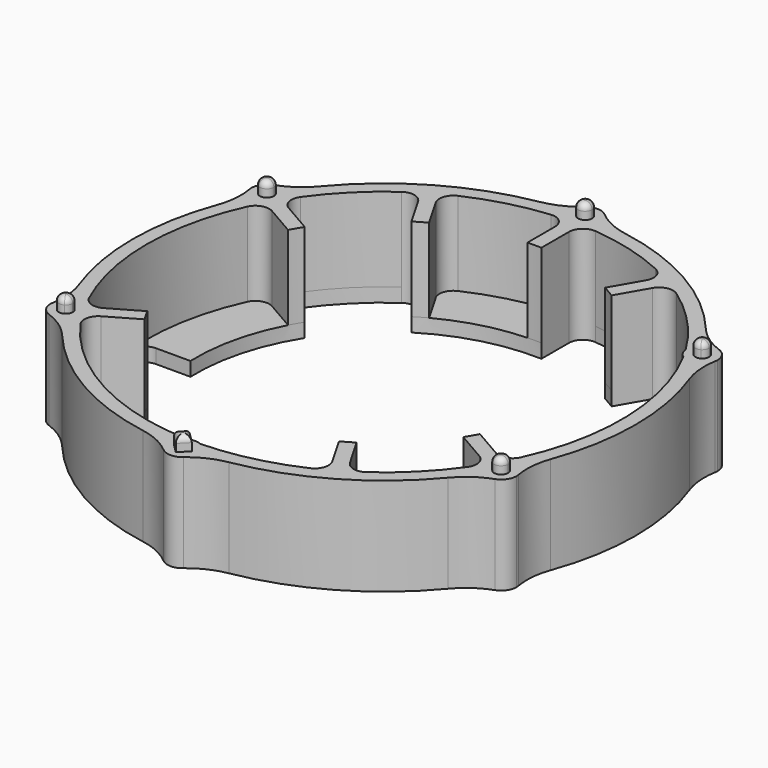
from build123d import *

# Parameters (mm, degrees)
F1_R         = 18
F1_R_2       = 17
F2_DEPTH     = 7
F3_DEPTH     = 7
F4_DEPTH     = 1
F6_DEPTH     = 7
F7_R         = 1
F8_R         = 5
F9_DEPTH     = 8
F10_R        = 0.44999
F11_DEPTH    = 1.8
F12_R        = 13.47
F13_DEPTH    = 1
F14_DEPTH    = 1
F15_T1_DEPTH = 1
F15_T3_DEPTH = 3.7395798703


# Not quite as in the source:
# - a fillet or chamfer that OpenCascade refuses, or shapes differently, is made with other operations: its cross-section is extruded or revolved along the edge and cut away or added
# - a fillet or chamfer is up to 0.001 mm smaller than in the source, because OpenCascade refuses the exact size


with BuildPart() as f2:
    # F1 (on Top) → F2 (new body)
    with BuildSketch(Plane.XY):
        Circle(F1_R)
        Circle(F1_R_2, mode=Mode.SUBTRACT)
    extrude(amount=F2_DEPTH)

    # F0 (on Top) → F3 (join)
    with BuildSketch(Plane.XY):
        with BuildLine():
            Line((-11.4073228059, 7.1633711619), (-14.4660626528, 8.9293354359))
            ThreePointArc((-14.4660626528, 8.9293354359), (-14.7224318643, 8.5), (-14.9660626528, 8.0633100321))
            Line((-14.9660626528, 8.0633100321), (-11.9073228059, 6.2973457581))
            ThreePointArc((-11.9073228059, 6.2973457581), (-11.665362189, 6.735), (-11.4073228059, 7.1633711619))
        make_face()
        with BuildLine():
            Line((7.1633711619, 11.4073228059), (8.9293354359, 14.4660626528))
            ThreePointArc((8.9293354359, 14.4660626528), (8.5, 14.7224318643), (8.0633100321, 14.9660626528))
            Line((8.0633100321, 14.9660626528), (6.2973457581, 11.9073228059))
            ThreePointArc((6.2973457581, 11.9073228059), (6.735, 11.665362189), (7.1633711619, 11.4073228059))
        make_face()
        with BuildLine():
            ThreePointArc((-14.9660626528, -8.0633100321), (-14.7224318643, -8.5), (-14.4660626528, -8.9293354359))
            Line((-14.4660626528, -8.9293354359), (-11.4073228059, -7.1633711619))
            ThreePointArc((-11.4073228059, -7.1633711619), (-11.665362189, -6.735), (-11.9073228059, -6.2973457581))
            Line((-11.9073228059, -6.2973457581), (-14.9660626528, -8.0633100321))
        make_face()
        with BuildLine():
            Line((-6.2973457581, 11.9073228059), (-8.0633100321, 14.9660626528))
            ThreePointArc((-8.0633100321, 14.9660626528), (-8.5, 14.7224318643), (-8.9293354359, 14.4660626528))
            Line((-8.9293354359, 14.4660626528), (-7.1633711619, 11.4073228059))
            ThreePointArc((-7.1633711619, 11.4073228059), (-6.735, 11.665362189), (-6.2973457581, 11.9073228059))
        make_face()
        with BuildLine():
            Line((0.5, 13.46071692), (0.5, 16.992645468))
            ThreePointArc((0.5, 16.992645468), (0, 17), (-0.5, 16.992645468))
            Line((-0.5, 16.992645468), (-0.5, 13.46071692))
            ThreePointArc((-0.5, 13.46071692), (0, 13.47), (0.5, 13.46071692))
        make_face()
        with BuildLine():
            ThreePointArc((14.4660626528, -8.9293354359), (14.7224318643, -8.5), (14.9660626528, -8.0633100321))
            Line((14.9660626528, -8.0633100321), (11.9073228059, -6.2973457581))
            ThreePointArc((11.9073228059, -6.2973457581), (11.665362189, -6.735), (11.4073228059, -7.1633711619))
            Line((11.4073228059, -7.1633711619), (14.4660626528, -8.9293354359))
        make_face()
        with BuildLine():
            ThreePointArc((8.0633100321, -14.9660626528), (8.5, -14.7224318643), (8.9293354359, -14.4660626528))
            Line((8.9293354359, -14.4660626528), (7.1633711619, -11.4073228059))
            ThreePointArc((7.1633711619, -11.4073228059), (6.735, -11.665362189), (6.2973457581, -11.9073228059))
            Line((6.2973457581, -11.9073228059), (8.0633100321, -14.9660626528))
        make_face()
    extrude(amount=F3_DEPTH)

    # F1 (on Top) → F4 (join)
    with BuildSketch(Plane.XY):
        Circle(F1_R)
        Circle(F1_R_2, mode=Mode.SUBTRACT)
        Circle(F1_R_2)
    extrude(amount=F4_DEPTH)

    # F5 (on Top) → F6 (join)
    with BuildSketch(Plane.XY):
        with BuildLine():
            ThreePointArc((-14.4884572681, 9), (-14.6275367743, 9.5353800561), (-15.0096060035, 9.935377578))
            ThreePointArc((-15.0096060035, 9.935377578), (-15.1731450826, 9.6837837802), (-15.3324673166, 9.4294987133))
            ThreePointArc((-15.3324673166, 9.4294987133), (-15.153718855, 9.2469868663), (-15.0884572681, 9))
            ThreePointArc((-15.0884572681, 9), (-15.3354561915, 8.5687338928), (-15.832419089, 8.5635568422))
            ThreePointArc((-15.832419089, 8.5635568422), (-15.9729752997, 8.2984372068), (-16.1090923805, 8.0310113108))
            ThreePointArc((-16.1090923805, 8.0310113108), (-15.0239657375, 8.0558870238), (-14.4884572681, 9))
        make_face()
        with BuildLine():
            ThreePointArc((-15.3324673166, 9.4294987133), (-15.1731450826, 9.6837837802), (-15.0096060035, 9.935377578))
            ThreePointArc((-15.0096060035, 9.935377578), (-16.5410852123, 9.55), (-16.1090923805, 8.0310113108))
            ThreePointArc((-16.1090923805, 8.0310113108), (-15.9729752997, 8.2984372068), (-15.832419089, 8.5635568422))
            ThreePointArc((-15.832419089, 8.5635568422), (-16.02146997, 9.25), (-15.3324673166, 9.4294987133))
        make_face()
        with BuildLine():
            ThreePointArc((-1.099486377, 17.9663888889), (0, 16.9), (1.099486377, 17.9663888889))
            ThreePointArc((1.099486377, 17.9663888889), (0.7998302171, 17.982220987), (0.4999517724, 17.9930555556))
            ThreePointArc((0.4999517724, 17.9930555556), (0, 17.5), (-0.4999517724, 17.9930555556))
            ThreePointArc((-0.4999517724, 17.9930555556), (-0.7998302171, 17.982220987), (-1.099486377, 17.9663888889))
        make_face()
        with BuildLine():
            ThreePointArc((0.4999517724, 17.9930555556), (0.7998302171, 17.982220987), (1.099486377, 17.9663888889))
            ThreePointArc((1.099486377, 17.9663888889), (1.0998715868, 17.9831924823), (1.1, 18))
            ThreePointArc((1.1, 18), (-0.0168075177, 19.0998715868), (-1.099486377, 17.9663888889))
            ThreePointArc((-1.099486377, 17.9663888889), (-0.7998302171, 17.982220987), (-0.4999517724, 17.9930555556))
            ThreePointArc((-0.4999517724, 17.9930555556), (-0.003472306, 18.4999879429), (0.5, 18))
            ThreePointArc((0.5, 18), (0.4999879429, 17.996527694), (0.4999517724, 17.9930555556))
        make_face()
        with BuildLine():
            ThreePointArc((15.832419089, 8.5635568422), (15.9729752997, 8.2984372068), (16.1090923805, 8.0310113108))
            ThreePointArc((16.1090923805, 8.0310113108), (16.5325702443, 8.4355084694), (16.6884572681, 9))
            ThreePointArc((16.6884572681, 9), (16.1238373242, 9.9609204939), (15.0096060035, 9.935377578))
            ThreePointArc((15.0096060035, 9.935377578), (15.1731450826, 9.6837837802), (15.3324673166, 9.4294987133))
            ThreePointArc((15.3324673166, 9.4294987133), (15.8354441344, 9.4347384132), (16.0884572681, 9))
            ThreePointArc((16.0884572681, 9), (16.0197233753, 8.7469989234), (15.832419089, 8.5635568422))
        make_face()
        with BuildLine():
            ThreePointArc((15.0096060035, 9.935377578), (14.635829324, 8.45), (16.1090923805, 8.0310113108))
            ThreePointArc((16.1090923805, 8.0310113108), (15.9729752997, 8.2984372068), (15.832419089, 8.5635568422))
            ThreePointArc((15.832419089, 8.5635568422), (15.1554445662, 8.75), (15.3324673166, 9.4294987133))
            ThreePointArc((15.3324673166, 9.4294987133), (15.1731450826, 9.6837837802), (15.0096060035, 9.935377578))
        make_face()
        with BuildLine():
            ThreePointArc((-15.3324673166, -9.4294987133), (-15.1731450826, -9.6837837802), (-15.0096060035, -9.935377578))
            ThreePointArc((-15.0096060035, -9.935377578), (-14.6275367743, -9.5353800561), (-14.4884572681, -9))
            ThreePointArc((-14.4884572681, -9), (-15.0239657375, -8.0558870238), (-16.1090923805, -8.0310113108))
            ThreePointArc((-16.1090923805, -8.0310113108), (-15.9729752997, -8.2984372068), (-15.832419089, -8.5635568422))
            ThreePointArc((-15.832419089, -8.5635568422), (-15.3354561915, -8.5687338928), (-15.0884572681, -9))
            ThreePointArc((-15.0884572681, -9), (-15.153718855, -9.2469868663), (-15.3324673166, -9.4294987133))
        make_face()
        with BuildLine():
            ThreePointArc((-16.1090923805, -8.0310113108), (-16.5410852123, -9.55), (-15.0096060035, -9.935377578))
            ThreePointArc((-15.0096060035, -9.935377578), (-15.1731450826, -9.6837837802), (-15.3324673166, -9.4294987133))
            ThreePointArc((-15.3324673166, -9.4294987133), (-16.02146997, -9.25), (-15.832419089, -8.5635568422))
            ThreePointArc((-15.832419089, -8.5635568422), (-15.9729752997, -8.2984372068), (-16.1090923805, -8.0310113108))
        make_face()
        with BuildLine():
            ThreePointArc((0.6255239257, -17.9891278226), (0.8625800837, -17.9793202207), (1.099486377, -17.9663888889))
            ThreePointArc((1.099486377, -17.9663888889), (0, -16.9), (-1.099486377, -17.9663888889))
            ThreePointArc((-1.099486377, -17.9663888889), (-0.8625800837, -17.9793202207), (-0.6255239257, -17.9891278226))
            Line((-0.6255239257, -17.9891278226), (0, -17.3636038969))
            Line((0, -17.3636038969), (0.6255239257, -17.9891278226))
        make_face()
        with BuildLine():
            ThreePointArc((1.1, -18), (1.0998715868, -17.9831924823), (1.099486377, -17.9663888889))
            ThreePointArc((1.099486377, -17.9663888889), (0.8625800837, -17.9793202207), (0.6255239257, -17.9891278226))
            Line((0.6255239257, -17.9891278226), (0.6363961031, -18))
            Line((0.6363961031, -18), (0, -18.6363961031))
            Line((0, -18.6363961031), (-0.6363961031, -18))
            Line((-0.6363961031, -18), (-0.6255239257, -17.9891278226))
            ThreePointArc((-0.6255239257, -17.9891278226), (-0.8625800837, -17.9793202207), (-1.099486377, -17.9663888889))
            ThreePointArc((-1.099486377, -17.9663888889), (-0.0168075177, -19.0998715868), (1.1, -18))
        make_face()
        with BuildLine():
            ThreePointArc((16.6884572681, -9), (16.5325702443, -8.4355084694), (16.1090923805, -8.0310113108))
            ThreePointArc((16.1090923805, -8.0310113108), (15.9729752997, -8.2984372068), (15.832419089, -8.5635568422))
            ThreePointArc((15.832419089, -8.5635568422), (16.0197233753, -8.7469989234), (16.0884572681, -9))
            ThreePointArc((16.0884572681, -9), (15.8354441344, -9.4347384132), (15.3324673166, -9.4294987133))
            ThreePointArc((15.3324673166, -9.4294987133), (15.1731450826, -9.6837837802), (15.0096060035, -9.935377578))
            ThreePointArc((15.0096060035, -9.935377578), (16.1238373242, -9.9609204939), (16.6884572681, -9))
        make_face()
        with BuildLine():
            ThreePointArc((15.832419089, -8.5635568422), (15.9729752997, -8.2984372068), (16.1090923805, -8.0310113108))
            ThreePointArc((16.1090923805, -8.0310113108), (14.635829324, -8.45), (15.0096060035, -9.935377578))
            ThreePointArc((15.0096060035, -9.935377578), (15.1731450826, -9.6837837802), (15.3324673166, -9.4294987133))
            ThreePointArc((15.3324673166, -9.4294987133), (15.1554445662, -8.75), (15.832419089, -8.5635568422))
        make_face()
        with BuildLine():
            ThreePointArc((-15.0884572681, 9), (-15.153718855, 9.2469868663), (-15.3324673166, 9.4294987133))
            ThreePointArc((-15.3324673166, 9.4294987133), (-15.5884572681, 9), (-15.832419089, 8.5635568422))
            ThreePointArc((-15.832419089, 8.5635568422), (-15.3354561915, 8.5687338928), (-15.0884572681, 9))
        make_face()
        with BuildLine():
            ThreePointArc((-15.832419089, 8.5635568422), (-15.5884572681, 9), (-15.3324673166, 9.4294987133))
            ThreePointArc((-15.3324673166, 9.4294987133), (-16.02146997, 9.25), (-15.832419089, 8.5635568422))
        make_face()
        with BuildLine():
            ThreePointArc((-0.4999517724, 17.9930555556), (0, 18), (0.4999517724, 17.9930555556))
            ThreePointArc((0.4999517724, 17.9930555556), (0.4999879429, 17.996527694), (0.5, 18))
            ThreePointArc((0.5, 18), (-0.003472306, 18.4999879429), (-0.4999517724, 17.9930555556))
        make_face()
        with BuildLine():
            ThreePointArc((-0.4999517724, 17.9930555556), (0, 17.5), (0.4999517724, 17.9930555556))
            ThreePointArc((0.4999517724, 17.9930555556), (0, 18), (-0.4999517724, 17.9930555556))
        make_face()
        with BuildLine():
            ThreePointArc((15.3324673166, 9.4294987133), (15.5884572681, 9), (15.832419089, 8.5635568422))
            ThreePointArc((15.832419089, 8.5635568422), (16.0197233753, 8.7469989234), (16.0884572681, 9))
            ThreePointArc((16.0884572681, 9), (15.8354441344, 9.4347384132), (15.3324673166, 9.4294987133))
        make_face()
        with BuildLine():
            ThreePointArc((15.3324673166, 9.4294987133), (15.1554445662, 8.75), (15.832419089, 8.5635568422))
            ThreePointArc((15.832419089, 8.5635568422), (15.5884572681, 9), (15.3324673166, 9.4294987133))
        make_face()
        with BuildLine():
            ThreePointArc((16.0884572681, -9), (16.0197233753, -8.7469989234), (15.832419089, -8.5635568422))
            ThreePointArc((15.832419089, -8.5635568422), (15.5884572681, -9), (15.3324673166, -9.4294987133))
            ThreePointArc((15.3324673166, -9.4294987133), (15.8354441344, -9.4347384132), (16.0884572681, -9))
        make_face()
        with BuildLine():
            ThreePointArc((15.3324673166, -9.4294987133), (15.5884572681, -9), (15.832419089, -8.5635568422))
            ThreePointArc((15.832419089, -8.5635568422), (15.1554445662, -8.75), (15.3324673166, -9.4294987133))
        make_face()
        with BuildLine():
            Line((0.6363961031, -18), (0.6255239257, -17.9891278226))
            ThreePointArc((0.6255239257, -17.9891278226), (0, -18), (-0.6255239257, -17.9891278226))
            Line((-0.6255239257, -17.9891278226), (-0.6363961031, -18))
            Line((-0.6363961031, -18), (0, -18.6363961031))
            Line((0, -18.6363961031), (0.6363961031, -18))
        make_face()
        with BuildLine():
            ThreePointArc((-15.832419089, -8.5635568422), (-16.02146997, -9.25), (-15.3324673166, -9.4294987133))
            ThreePointArc((-15.3324673166, -9.4294987133), (-15.5884572681, -9), (-15.832419089, -8.5635568422))
        make_face()
        with BuildLine():
            ThreePointArc((-15.832419089, -8.5635568422), (-15.5884572681, -9), (-15.3324673166, -9.4294987133))
            ThreePointArc((-15.3324673166, -9.4294987133), (-15.153718855, -9.2469868663), (-15.0884572681, -9))
            ThreePointArc((-15.0884572681, -9), (-15.3354561915, -8.5687338928), (-15.832419089, -8.5635568422))
        make_face()
        with BuildLine():
            ThreePointArc((-0.6255239257, -17.9891278226), (0, -18), (0.6255239257, -17.9891278226))
            Line((0.6255239257, -17.9891278226), (0, -17.3636038969))
            Line((0, -17.3636038969), (-0.6255239257, -17.9891278226))
        make_face()
    extrude(amount=F6_DEPTH)

    # F7
    f7_edges = [f2.edges().sort_by_distance(p)[0] for p in [
        (0.5, 16.992645, 4),
        (8.06331, 14.966063, 4),
        (-14.966063, -8.06331, 4),
        (8.929335, -14.466063, 4),
        (14.966063, -8.06331, 4),
        (-0.5, 16.992645, 4),
        (-14.966063, 8.06331, 4),
        (-8.929335, 14.466063, 4),
        (-14.466063, 8.929335, 4),
        (-8.06331, 14.966063, 4),
        (-14.466063, -8.929335, 4),
        (8.929335, 14.466063, 4),
        (8.06331, -14.966063, 4),
        (14.466063, -8.929335, 4),
    ]]
    fillet(f7_edges, radius=F7_R)

    # F8 (call 1 of 12: OpenCascade refuses the feature's edges together)
    f8_edges = [f2.edges().sort_by_distance(p)[0] for p in [
        (-16.109092, 8.031011, 3.5),
    ]]
    fillet(f8_edges, radius=F8_R)

    # F8#2 (call 2 of 12)
    f8_2_edges = [f2.edges().sort_by_distance(p)[0] for p in [
        (-15.009606, 9.935378, 3.5),
    ]]
    fillet(f8_2_edges, radius=F8_R)

    # F8#3 (call 3 of 12)
    f8_3_edges = [f2.edges().sort_by_distance(p)[0] for p in [
        (-1.099486, 17.966389, 3.5),
    ]]
    fillet(f8_3_edges, radius=F8_R)

    # F8#4 (call 4 of 12)
    f8_4_edges = [f2.edges().sort_by_distance(p)[0] for p in [
        (1.099486, 17.966389, 3.5),
    ]]
    fillet(f8_4_edges, radius=F8_R)

    # F8#5 (call 5 of 12)
    f8_5_edges = [f2.edges().sort_by_distance(p)[0] for p in [
        (-15.009606, -9.935378, 3.5),
    ]]
    fillet(f8_5_edges, radius=F8_R)

    # F8#6 (call 6 of 12)
    f8_6_edges = [f2.edges().sort_by_distance(p)[0] for p in [
        (-16.109092, -8.031011, 3.5),
    ]]
    fillet(f8_6_edges, radius=F8_R)

    # F8#7 (call 7 of 12)
    f8_7_edges = [f2.edges().sort_by_distance(p)[0] for p in [
        (1.099486, -17.966389, 3.5),
    ]]
    fillet(f8_7_edges, radius=F8_R)

    # F8#8 (call 8 of 12)
    f8_8_edges = [f2.edges().sort_by_distance(p)[0] for p in [
        (-1.099486, -17.966389, 3.5),
    ]]
    fillet(f8_8_edges, radius=F8_R)

    # F8#10 (call 9 of 12)
    f8_10_edges = [f2.edges().sort_by_distance(p)[0] for p in [
        (15.009606, -9.935378, 3.5),
    ]]
    fillet(f8_10_edges, radius=F8_R)

    # F8#11 (call 10 of 12)
    f8_11_edges = [f2.edges().sort_by_distance(p)[0] for p in [
        (16.109092, 8.031011, 3.5),
    ]]
    fillet(f8_11_edges, radius=F8_R)

    # F8#12 (call 11 of 12)
    f8_12_edges = [f2.edges().sort_by_distance(p)[0] for p in [
        (15.009606, 9.935378, 3.5),
    ]]
    fillet(f8_12_edges, radius=F8_R)

    # F8#9 (call 12 of 12)
    f8_9_edges = [f2.edges().sort_by_distance(p)[0] for p in [
        (16.109092, -8.031011, 3.5),
    ]]
    fillet(f8_9_edges, radius=F8_R)

    # F5 (on Top) → F9 (join)
    with BuildSketch(Plane.XY):
        with BuildLine():
            ThreePointArc((-15.832419089, 8.5635568422), (-15.5884572681, 9), (-15.3324673166, 9.4294987133))
            ThreePointArc((-15.3324673166, 9.4294987133), (-16.02146997, 9.25), (-15.832419089, 8.5635568422))
        make_face()
        with BuildLine():
            ThreePointArc((-15.0884572681, 9), (-15.153718855, 9.2469868663), (-15.3324673166, 9.4294987133))
            ThreePointArc((-15.3324673166, 9.4294987133), (-15.5884572681, 9), (-15.832419089, 8.5635568422))
            ThreePointArc((-15.832419089, 8.5635568422), (-15.3354561915, 8.5687338928), (-15.0884572681, 9))
        make_face()
        with BuildLine():
            ThreePointArc((-0.4999517724, 17.9930555556), (0, 18), (0.4999517724, 17.9930555556))
            ThreePointArc((0.4999517724, 17.9930555556), (0.4999879429, 17.996527694), (0.5, 18))
            ThreePointArc((0.5, 18), (-0.003472306, 18.4999879429), (-0.4999517724, 17.9930555556))
        make_face()
        with BuildLine():
            ThreePointArc((-0.4999517724, 17.9930555556), (0, 17.5), (0.4999517724, 17.9930555556))
            ThreePointArc((0.4999517724, 17.9930555556), (0, 18), (-0.4999517724, 17.9930555556))
        make_face()
        with BuildLine():
            ThreePointArc((15.3324673166, 9.4294987133), (15.1554445662, 8.75), (15.832419089, 8.5635568422))
            ThreePointArc((15.832419089, 8.5635568422), (15.5884572681, 9), (15.3324673166, 9.4294987133))
        make_face()
        with BuildLine():
            ThreePointArc((15.3324673166, 9.4294987133), (15.5884572681, 9), (15.832419089, 8.5635568422))
            ThreePointArc((15.832419089, 8.5635568422), (16.0197233753, 8.7469989234), (16.0884572681, 9))
            ThreePointArc((16.0884572681, 9), (15.8354441344, 9.4347384132), (15.3324673166, 9.4294987133))
        make_face()
        with BuildLine():
            ThreePointArc((15.3324673166, -9.4294987133), (15.5884572681, -9), (15.832419089, -8.5635568422))
            ThreePointArc((15.832419089, -8.5635568422), (15.1554445662, -8.75), (15.3324673166, -9.4294987133))
        make_face()
        with BuildLine():
            ThreePointArc((16.0884572681, -9), (16.0197233753, -8.7469989234), (15.832419089, -8.5635568422))
            ThreePointArc((15.832419089, -8.5635568422), (15.5884572681, -9), (15.3324673166, -9.4294987133))
            ThreePointArc((15.3324673166, -9.4294987133), (15.8354441344, -9.4347384132), (16.0884572681, -9))
        make_face()
        with BuildLine():
            Line((0.6363961031, -18), (0.6255239257, -17.9891278226))
            ThreePointArc((0.6255239257, -17.9891278226), (0, -18), (-0.6255239257, -17.9891278226))
            Line((-0.6255239257, -17.9891278226), (-0.6363961031, -18))
            Line((-0.6363961031, -18), (0, -18.6363961031))
            Line((0, -18.6363961031), (0.6363961031, -18))
        make_face()
        with BuildLine():
            ThreePointArc((-0.6255239257, -17.9891278226), (0, -18), (0.6255239257, -17.9891278226))
            Line((0.6255239257, -17.9891278226), (0, -17.3636038969))
            Line((0, -17.3636038969), (-0.6255239257, -17.9891278226))
        make_face()
        with BuildLine():
            ThreePointArc((-15.832419089, -8.5635568422), (-16.02146997, -9.25), (-15.3324673166, -9.4294987133))
            ThreePointArc((-15.3324673166, -9.4294987133), (-15.5884572681, -9), (-15.832419089, -8.5635568422))
        make_face()
        with BuildLine():
            ThreePointArc((-15.832419089, -8.5635568422), (-15.5884572681, -9), (-15.3324673166, -9.4294987133))
            ThreePointArc((-15.3324673166, -9.4294987133), (-15.153718855, -9.2469868663), (-15.0884572681, -9))
            ThreePointArc((-15.0884572681, -9), (-15.3354561915, -8.5687338928), (-15.832419089, -8.5635568422))
        make_face()
    extrude(amount=F9_DEPTH)

    # F10 (radius 0.45 in the source; OpenCascade refuses exactly that, so slightly less here)
    f10_edges = [f2.edges().sort_by_distance(p)[0] for p in [
        (-15.844447, -8.570501, 8),
        (-15.344495, 9.436443, 8),
        (0.499952, 18.006944, 8),
        (15.344495, 9.436443, 8),
        (15.844447, -8.570501, 8),
        (0.318198, -17.681802, 8),
        (-0.318198, -18.318198, 8),
        (0.318198, -18.318198, 8),
        (-0.318198, -17.681802, 8),
    ]]
    fillet(f10_edges, radius=F10_R)

    # F5 (on Top) → F11 (cut)
    with BuildSketch(Plane.XY):
        with BuildLine():
            ThreePointArc((-15.832419089, -8.5635568422), (-16.02146997, -9.25), (-15.3324673166, -9.4294987133))
            ThreePointArc((-15.3324673166, -9.4294987133), (-15.5884572681, -9), (-15.832419089, -8.5635568422))
        make_face()
        with BuildLine():
            ThreePointArc((-15.832419089, -8.5635568422), (-15.5884572681, -9), (-15.3324673166, -9.4294987133))
            ThreePointArc((-15.3324673166, -9.4294987133), (-15.153718855, -9.2469868663), (-15.0884572681, -9))
            ThreePointArc((-15.0884572681, -9), (-15.3354561915, -8.5687338928), (-15.832419089, -8.5635568422))
        make_face()
        with BuildLine():
            Line((0.6363961031, -18), (0.6255239257, -17.9891278226))
            ThreePointArc((0.6255239257, -17.9891278226), (0, -18), (-0.6255239257, -17.9891278226))
            Line((-0.6255239257, -17.9891278226), (-0.6363961031, -18))
            Line((-0.6363961031, -18), (0, -18.6363961031))
            Line((0, -18.6363961031), (0.6363961031, -18))
        make_face()
        with BuildLine():
            ThreePointArc((-0.6255239257, -17.9891278226), (0, -18), (0.6255239257, -17.9891278226))
            Line((0.6255239257, -17.9891278226), (0, -17.3636038969))
            Line((0, -17.3636038969), (-0.6255239257, -17.9891278226))
        make_face()
        with BuildLine():
            ThreePointArc((15.3324673166, -9.4294987133), (15.5884572681, -9), (15.832419089, -8.5635568422))
            ThreePointArc((15.832419089, -8.5635568422), (15.1554445662, -8.75), (15.3324673166, -9.4294987133))
        make_face()
        with BuildLine():
            ThreePointArc((16.0884572681, -9), (16.0197233753, -8.7469989234), (15.832419089, -8.5635568422))
            ThreePointArc((15.832419089, -8.5635568422), (15.5884572681, -9), (15.3324673166, -9.4294987133))
            ThreePointArc((15.3324673166, -9.4294987133), (15.8354441344, -9.4347384132), (16.0884572681, -9))
        make_face()
        with BuildLine():
            ThreePointArc((15.3324673166, 9.4294987133), (15.1554445662, 8.75), (15.832419089, 8.5635568422))
            ThreePointArc((15.832419089, 8.5635568422), (15.5884572681, 9), (15.3324673166, 9.4294987133))
        make_face()
        with BuildLine():
            ThreePointArc((15.3324673166, 9.4294987133), (15.5884572681, 9), (15.832419089, 8.5635568422))
            ThreePointArc((15.832419089, 8.5635568422), (16.0197233753, 8.7469989234), (16.0884572681, 9))
            ThreePointArc((16.0884572681, 9), (15.8354441344, 9.4347384132), (15.3324673166, 9.4294987133))
        make_face()
        with BuildLine():
            ThreePointArc((-0.4999517724, 17.9930555556), (0, 17.5), (0.4999517724, 17.9930555556))
            ThreePointArc((0.4999517724, 17.9930555556), (0, 18), (-0.4999517724, 17.9930555556))
        make_face()
        with BuildLine():
            ThreePointArc((-0.4999517724, 17.9930555556), (0, 18), (0.4999517724, 17.9930555556))
            ThreePointArc((0.4999517724, 17.9930555556), (0.4999879429, 17.996527694), (0.5, 18))
            ThreePointArc((0.5, 18), (-0.003472306, 18.4999879429), (-0.4999517724, 17.9930555556))
        make_face()
        with BuildLine():
            ThreePointArc((-15.832419089, 8.5635568422), (-15.5884572681, 9), (-15.3324673166, 9.4294987133))
            ThreePointArc((-15.3324673166, 9.4294987133), (-16.02146997, 9.25), (-15.832419089, 8.5635568422))
        make_face()
        with BuildLine():
            ThreePointArc((-15.0884572681, 9), (-15.153718855, 9.2469868663), (-15.3324673166, 9.4294987133))
            ThreePointArc((-15.3324673166, 9.4294987133), (-15.5884572681, 9), (-15.832419089, 8.5635568422))
            ThreePointArc((-15.832419089, 8.5635568422), (-15.3354561915, 8.5687338928), (-15.0884572681, 9))
        make_face()
    extrude(amount=F11_DEPTH, mode=Mode.SUBTRACT)

    # F12 (on Top) → F13 (cut)
    with BuildSketch(Plane.XY):
        Circle(F12_R)
    extrude(amount=F13_DEPTH, mode=Mode.SUBTRACT)

    # F0 (on Top) → F14 (cut)
    with BuildSketch(Plane.XY):
        with BuildLine():
            ThreePointArc((0.5, -16.992645468), (4.3999237667, -16.4207390469), (8.0633100321, -14.9660626528))
            Line((8.0633100321, -14.9660626528), (6.2973457581, -11.9073228059))
            ThreePointArc((6.2973457581, -11.9073228059), (3.4862925375, -13.0110208801), (0.5, -13.46071692))
            Line((0.5, -13.46071692), (0.5, -16.992645468))
        make_face()
        with BuildLine():
            ThreePointArc((8.9293354359, -14.4660626528), (12.0208152802, -12.0208152802), (14.4660626528, -8.9293354359))
            Line((14.4660626528, -8.9293354359), (11.4073228059, -7.1633711619))
            ThreePointArc((11.4073228059, -7.1633711619), (9.5247283426, -9.5247283426), (7.1633711619, -11.4073228059))
            Line((7.1633711619, -11.4073228059), (8.9293354359, -14.4660626528))
        make_face()
        with BuildLine():
            Line((13.46071692, 0.5), (16.992645468, 0.5))
            ThreePointArc((16.992645468, 0.5), (16.4207390469, 4.3999237667), (14.9660626528, 8.0633100321))
            Line((14.9660626528, 8.0633100321), (11.9073228059, 6.2973457581))
            ThreePointArc((11.9073228059, 6.2973457581), (13.0110208801, 3.4862925375), (13.46071692, 0.5))
        make_face()
        with BuildLine():
            Line((11.4073228059, 7.1633711619), (14.4660626528, 8.9293354359))
            ThreePointArc((14.4660626528, 8.9293354359), (12.0208152802, 12.0208152802), (8.9293354359, 14.4660626528))
            Line((8.9293354359, 14.4660626528), (7.1633711619, 11.4073228059))
            ThreePointArc((7.1633711619, 11.4073228059), (9.5247283426, 9.5247283426), (11.4073228059, 7.1633711619))
        make_face()
        with BuildLine():
            Line((6.2973457581, 11.9073228059), (8.0633100321, 14.9660626528))
            ThreePointArc((8.0633100321, 14.9660626528), (4.3999237667, 16.4207390469), (0.5, 16.992645468))
            Line((0.5, 16.992645468), (0.5, 13.46071692))
            ThreePointArc((0.5, 13.46071692), (3.4862925375, 13.0110208801), (6.2973457581, 11.9073228059))
        make_face()
        with BuildLine():
            Line((-7.1633711619, 11.4073228059), (-8.9293354359, 14.4660626528))
            ThreePointArc((-8.9293354359, 14.4660626528), (-12.0208152802, 12.0208152802), (-14.4660626528, 8.9293354359))
            Line((-14.4660626528, 8.9293354359), (-11.4073228059, 7.1633711619))
            ThreePointArc((-11.4073228059, 7.1633711619), (-9.5247283426, 9.5247283426), (-7.1633711619, 11.4073228059))
        make_face()
        with BuildLine():
            ThreePointArc((-16.992645468, -0.5), (-16.4207390469, -4.3999237667), (-14.9660626528, -8.0633100321))
            Line((-14.9660626528, -8.0633100321), (-11.9073228059, -6.2973457581))
            ThreePointArc((-11.9073228059, -6.2973457581), (-13.0110208801, -3.4862925375), (-13.46071692, -0.5))
            Line((-13.46071692, -0.5), (-16.992645468, -0.5))
        make_face()
        with BuildLine():
            ThreePointArc((-14.4660626528, -8.9293354359), (-12.0208152802, -12.0208152802), (-8.9293354359, -14.4660626528))
            Line((-8.9293354359, -14.4660626528), (-7.1633711619, -11.4073228059))
            ThreePointArc((-7.1633711619, -11.4073228059), (-9.5247283426, -9.5247283426), (-11.4073228059, -7.1633711619))
            Line((-11.4073228059, -7.1633711619), (-14.4660626528, -8.9293354359))
        make_face()
    extrude(amount=F14_DEPTH, mode=Mode.SUBTRACT)

    # F15: fillet of radius 1 on 16 edges, made by hand

    # F15_s2 → F15_t1 (join)
    with BuildSketch(Plane.XY):
        with BuildLine():
            ThreePointArc((-16.9251280922, -1.59375), (-16.669042295, -0.8268543991), (-15.9295323221, -0.5))
            Line((-15.9295323221, -0.5), (-16.992645468, -0.5))
            ThreePointArc((-16.992645468, -0.5), (-16.9677020567, -1.0474191685), (-16.9251280922, -1.59375))
        make_face()
        with BuildLine():
            ThreePointArc((-9.8427920334, -13.8607158902), (-9.0505980623, -14.0223868846), (-8.3977788629, -13.5453796613))
            Line((-8.3977788629, -13.5453796613), (-8.9293354359, -14.4660626528))
            ThreePointArc((-8.9293354359, -14.4660626528), (-9.3909426367, -14.1707514407), (-9.8427920334, -13.8607158902))
        make_face()
        with BuildLine():
            ThreePointArc((1.59375, -16.9251280922), (0.8268543991, -16.669042295), (0.5, -15.9295323221))
            Line((0.5, -15.9295323221), (0.5, -16.992645468))
            ThreePointArc((0.5, -16.992645468), (1.0474191685, -16.9677020567), (1.59375, -16.9251280922))
        make_face()
        with BuildLine():
            ThreePointArc((16.9251280922, 1.59375), (16.669042295, 0.8268543991), (15.9295323221, 0.5))
            Line((15.9295323221, 0.5), (16.992645468, 0.5))
            ThreePointArc((16.992645468, 0.5), (16.9677020567, 1.0474191685), (16.9251280922, 1.59375))
        make_face()
        with BuildLine():
            ThreePointArc((13.8607158902, 9.8427920334), (14.0223868846, 9.0505980623), (13.5453796613, 8.3977788629))
            Line((13.5453796613, 8.3977788629), (14.4660626528, 8.9293354359))
            ThreePointArc((14.4660626528, 8.9293354359), (14.1707514407, 9.3909426367), (13.8607158902, 9.8427920334))
        make_face()
        with BuildLine():
            ThreePointArc((15.4544658902, 7.0823360588), (14.8492412837, 7.6184442326), (14.0453796613, 7.5317534591))
            Line((14.0453796613, 7.5317534591), (14.9660626528, 8.0633100321))
            ThreePointArc((14.9660626528, 8.0633100321), (15.2181706092, 7.57675942), (15.4544658902, 7.0823360588))
        make_face()
    extrude(amount=F15_T1_DEPTH)

    # F15_s4 → F15_t3 (join)
    with BuildSketch(Plane.XY):
        with BuildLine():
            ThreePointArc((-13.8607158902, -9.8427920334), (-14.0223868846, -9.0505980623), (-13.5453796613, -8.3977788629))
            Line((-13.5453796613, -8.3977788629), (-14.4660626528, -8.9293354359))
            ThreePointArc((-14.4660626528, -8.9293354359), (-14.1707514407, -9.3909426367), (-13.8607158902, -9.8427920334))
        make_face()
        with BuildLine():
            ThreePointArc((-13.5453796613, 8.3977788629), (-14.0223868846, 9.0505980623), (-13.8607158902, 9.8427920334))
            ThreePointArc((-13.8607158902, 9.8427920334), (-14.1707514407, 9.3909426367), (-14.4660626528, 8.9293354359))
            Line((-14.4660626528, 8.9293354359), (-13.5453796613, 8.3977788629))
        make_face()
        with BuildLine():
            ThreePointArc((-14.0453796613, -7.5317534591), (-14.8492412838, -7.6184442326), (-15.4544658902, -7.0823360588))
            ThreePointArc((-15.4544658902, -7.0823360588), (-15.2181706092, -7.57675942), (-14.9660626528, -8.0633100321))
            Line((-14.9660626528, -8.0633100321), (-14.0453796613, -7.5317534591))
        make_face()
        with BuildLine():
            ThreePointArc((8.3977788629, -13.5453796613), (9.0505980623, -14.0223868846), (9.8427920334, -13.8607158902))
            ThreePointArc((9.8427920334, -13.8607158902), (9.3909426367, -14.1707514407), (8.9293354359, -14.4660626528))
            Line((8.9293354359, -14.4660626528), (8.3977788629, -13.5453796613))
        make_face()
        with BuildLine():
            ThreePointArc((7.5317534591, -14.0453796613), (7.6184442326, -14.8492412838), (7.0823360588, -15.4544658902))
            ThreePointArc((7.0823360588, -15.4544658902), (7.57675942, -15.2181706092), (8.0633100321, -14.9660626528))
            Line((8.0633100321, -14.9660626528), (7.5317534591, -14.0453796613))
        make_face()
        with BuildLine():
            ThreePointArc((7.5317534591, 14.0453796613), (7.6184442326, 14.8492412838), (7.0823360588, 15.4544658902))
            ThreePointArc((7.0823360588, 15.4544658902), (7.57675942, 15.2181706092), (8.0633100321, 14.9660626528))
            Line((8.0633100321, 14.9660626528), (7.5317534591, 14.0453796613))
        make_face()
        with BuildLine():
            ThreePointArc((1.59375, 16.9251280922), (0.8268543991, 16.669042295), (0.5, 15.9295323221))
            Line((0.5, 15.9295323221), (0.5, 16.992645468))
            ThreePointArc((0.5, 16.992645468), (1.0474191685, 16.9677020567), (1.59375, 16.9251280922))
        make_face()
        with BuildLine():
            ThreePointArc((-9.8427920334, 13.8607158902), (-9.0505980623, 14.0223868846), (-8.3977788629, 13.5453796613))
            Line((-8.3977788629, 13.5453796613), (-8.9293354359, 14.4660626528))
            ThreePointArc((-8.9293354359, 14.4660626528), (-9.3909426367, 14.1707514407), (-9.8427920334, 13.8607158902))
        make_face()
        with BuildLine():
            ThreePointArc((9.8427920334, 13.8607158902), (9.0505980623, 14.0223868846), (8.3977788629, 13.5453796613))
            Line((8.3977788629, 13.5453796613), (8.9293354359, 14.4660626528))
            ThreePointArc((8.9293354359, 14.4660626528), (9.3909426367, 14.1707514407), (9.8427920334, 13.8607158902))
        make_face()
        with BuildLine():
            ThreePointArc((13.8607158902, -9.8427920334), (14.0223868846, -9.0505980623), (13.5453796613, -8.3977788629))
            Line((13.5453796613, -8.3977788629), (14.4660626528, -8.9293354359))
            ThreePointArc((14.4660626528, -8.9293354359), (14.1707514407, -9.3909426367), (13.8607158902, -9.8427920334))
        make_face()
    extrude(amount=F15_T3_DEPTH)


solid = f2.part
